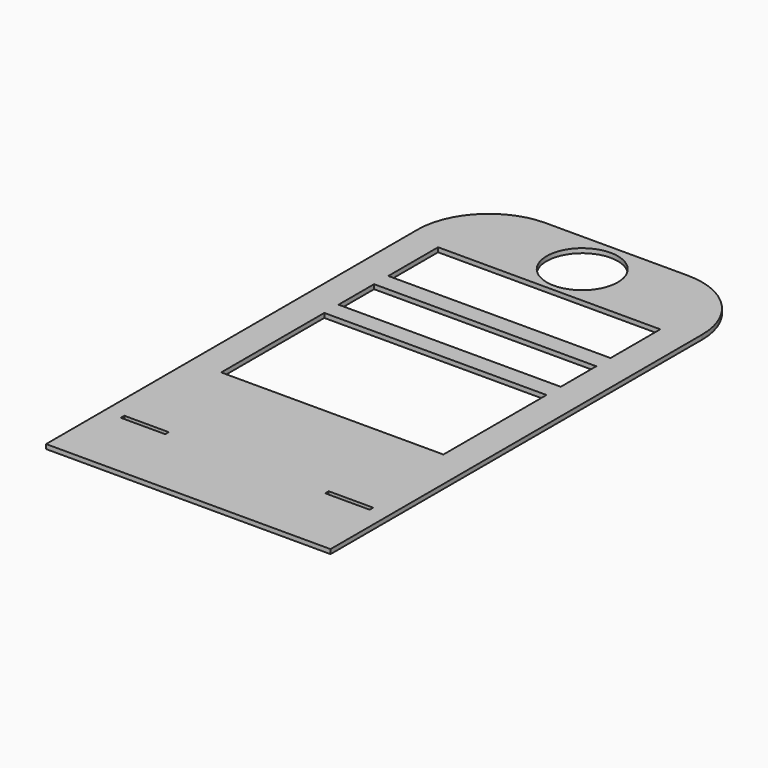
from build123d import *

# Parameters (mm, degrees)
F0_W     = 127
F0_H     = 12.7
F0_W_2   = 635
F0_H_2   = 126.9999911487
F0_R     = 101.6
F0_H_3   = 177.8000088513
F1_DEPTH = 12.7


# Not quite as in the source:
# - a feature names something its author has since deleted; it is built from what else it names


with BuildPart() as f1:
    # F0 (on Top) → F1 (new body)
    with BuildSketch(Plane.XY):
        with BuildLine():
            ThreePointArc((-444.8386187891, 967.019580251), (-588.5227167262, 907.5036781881), (-648.0386187891, 763.819580251))
            Line((-648.0386187891, 763.819580251), (-648.0386187891, -556.980419749))
            Line((-648.0386187891, -556.980419749), (-648.0386187891, -563.330419749))
            Line((-648.0386187891, -563.330419749), (164.7613812109, -563.330419749))
            Line((164.7613812109, -563.330419749), (164.7613812109, -556.980419749))
            Line((164.7613812109, -556.980419749), (164.7613812109, 763.819580251))
            ThreePointArc((164.7613812109, 763.819580251), (105.245479148, 907.5036781881), (-38.4386187891, 967.019580251))
            Line((-38.4386187891, 967.019580251), (-444.8386187891, 967.019580251))
        make_face()
        with Locations((-533.7386187891, -353.780419749)):
            Rectangle(F0_W, F0_H, mode=Mode.SUBTRACT)
        with Locations((50.4613812109, -353.780419749)):
            Rectangle(F0_W, F0_H, mode=Mode.SUBTRACT)
        Polygon((75.8613812109, -48.980419749), (-559.1386187891, -48.980419749), (-559.1386187891, 90.719580251), (-559.1386187891, 141.519580251), (-559.1386187891, 319.319580251), (75.8613812109, 319.319580251), (75.8613812109, 141.519580251), (75.8613812109, 90.719580251), align=None, mode=Mode.SUBTRACT)
        with Locations((-241.6386187891, 433.6195758253)):
            Rectangle(F0_W_2, F0_H_2, mode=Mode.SUBTRACT)
        with Locations((-241.6386187891, 843.8264727592)):
            Circle(F0_R, mode=Mode.SUBTRACT)
        with Locations((-241.6386187891, 636.8195758253)):
            Rectangle(F0_W_2, F0_H_3, mode=Mode.SUBTRACT)
    extrude(amount=F1_DEPTH)


solid = f1.part
